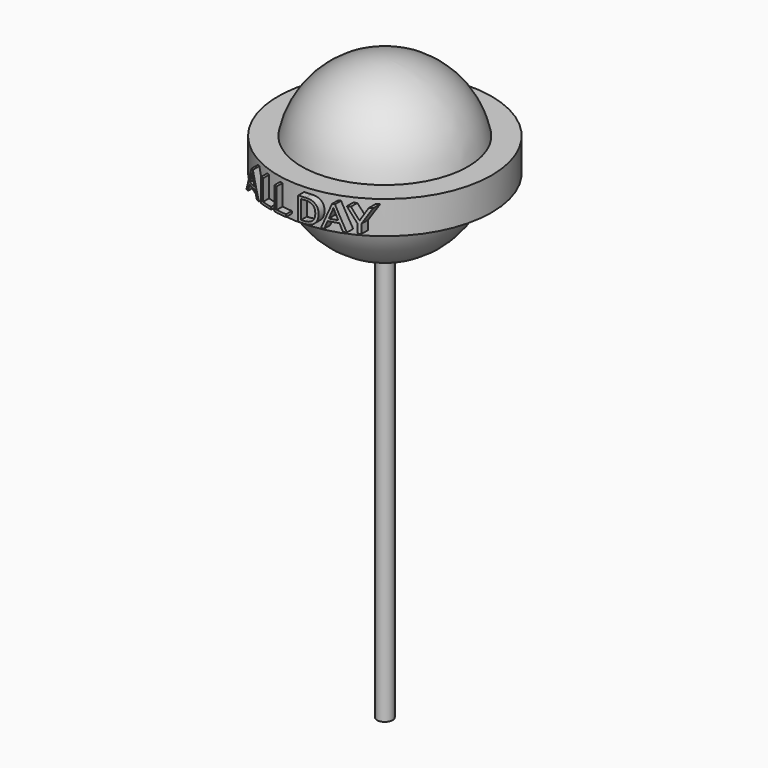
from build123d import *

# Parameters (mm, degrees)
F2_TEXT_SIZE = 6.7334366678
F3_DEPTH     = 28.5


# Not quite as in the source:
# - Text() gives the source's letters only with a copy of the font that has no kerning and outlines rounded to 1/6400 em; it was checked with that copy


with BuildPart() as f1:
    # F0 (on Front) → F1 (revolve)
    with BuildSketch(Plane.XZ):
        with BuildLine():
            Line((0, -15.00000339), (0, -17.5736437741))
            ThreePointArc((0, -17.5736437741), (0.804303768, -17.5552285929), (1.6069218982, -17.5000216432))
            Line((1.6069218982, -17.5000216432), (1.6069218982, -15.00000339))
            Line((1.6069218982, -15.00000339), (0, -15.00000339))
        make_face()
        with BuildLine():
            ThreePointArc((1.6069218982, -17.5000216432), (0.804303768, -17.5552285929), (0, -17.5736437741))
            Line((0, -17.5736437741), (0, -102.6785746217))
            Line((0, -102.6785746217), (1.6069218982, -102.6785746217))
            Line((1.6069218982, -102.6785746217), (1.6069218982, -17.5000216432))
        make_face()
        with BuildLine():
            Line((1.6069218982, -15.00000339), (1.6069218982, -17.5000216432))
            ThreePointArc((1.6069218982, -17.5000216432), (11.7721292476, -13.0479856099), (17.2430123548, -3.3928572666))
            Line((17.2430123548, -3.3928572666), (7.8571420163, -3.3928572666))
            Line((7.8571420163, -3.3928572666), (7.8571420163, 3.3928572666))
            Line((7.8571420163, 3.3928572666), (17.2430123548, 3.3928572666))
            ThreePointArc((17.2430123548, 3.3928572666), (11.1626182081, 13.5730950869), (0, 17.5736437741))
            Line((0, 17.5736437741), (0, -15.00000339))
            Line((0, -15.00000339), (1.6069218982, -15.00000339))
        make_face()
        with BuildLine():
            Line((7.8571420163, -3.3928572666), (17.2430123548, -3.3928572666))
            ThreePointArc((17.2430123548, -3.3928572666), (17.5736437741, 0), (17.2430123548, 3.3928572666))
            Line((17.2430123548, 3.3928572666), (7.8571420163, 3.3928572666))
            Line((7.8571420163, 3.3928572666), (7.8571420163, -3.3928572666))
        make_face()
        with BuildLine():
            ThreePointArc((17.2430123548, 3.3928572666), (17.5736437741, 0), (17.2430123548, -3.3928572666))
            Line((17.2430123548, -3.3928572666), (22.1428573132, -3.3928572666))
            Line((22.1428573132, -3.3928572666), (22.1428573132, 3.3928572666))
            Line((22.1428573132, 3.3928572666), (17.2430123548, 3.3928572666))
        make_face()
    revolve(axis=Axis((0, 0, 27.4107158184), (0, 0, 1)))

    # F2 (on Front) → F3 (join)
    with BuildSketch(Plane.XZ):
        with Locations((-12.7062099054, -2.3563660216)):
            Text('ALL DAY', F2_TEXT_SIZE, font='Open Sans', text_align=(TextAlign.LEFT, TextAlign.BOTTOM))
    extrude(amount=F3_DEPTH)

    # F4 (on Front) → F5 (revolve, cut)
    with BuildSketch(Plane.XZ):
        Polygon((23.6428573132, 4.8928572666), (23.6428573132, -4.8928572666), (18.05007644, -4.8928572666), (19.0970599651, -15.3208912686), (34.4652459025, -11.8808101267), (34.4652459025, 0.9821000407), (29.1181635112, 12.7719489262), (15.2082722634, 12.4728118405), (17.6013708115, 4.8928572666), align=None)
    revolve(axis=Axis((0, 0, 29.8852063715), (0, 0, 1)), mode=Mode.SUBTRACT)


solid = f1.part
